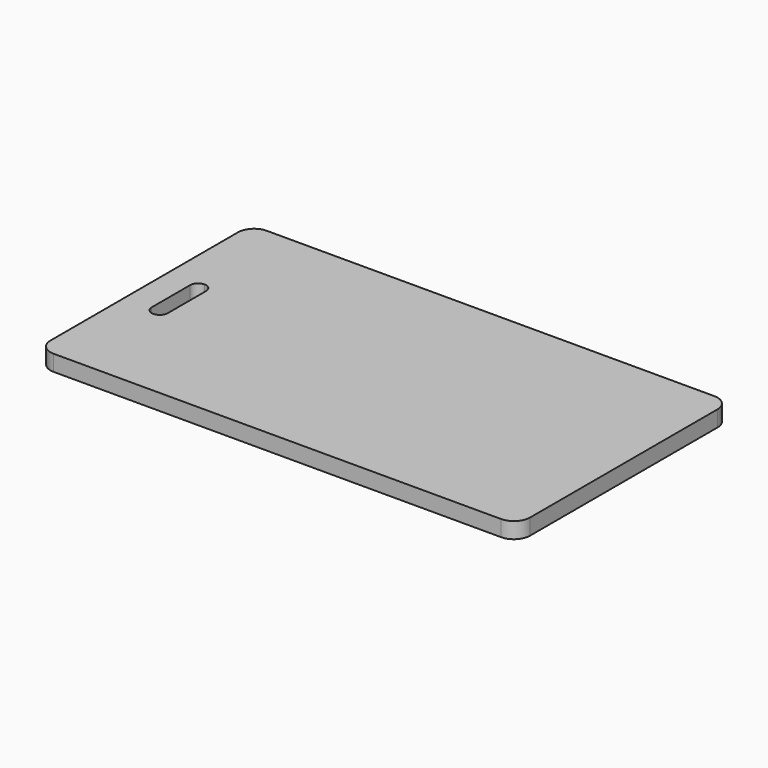
from build123d import *

# Parameters (mm, degrees)
F0_W     = 3
F0_H     = 12
F1_DEPTH = 3
F2_R     = 1.49999


# Not quite as in the source:
# - a fillet or chamfer is up to 0.001 mm smaller than in the source, because OpenCascade refuses the exact size
# - a feature of the source that left no trace in its solid (it failed there, or was rolled back) is left out


with BuildPart() as f1:
    # F0 (on Top) → F1 (new body)
    with BuildSketch(Plane.XY):
        with BuildLine():
            ThreePointArc((0, 3), (0.8786796564, 0.8786796564), (3, 0))
            Line((3, 0), (87, 0))
            ThreePointArc((87, 0), (89.1213203436, 0.8786796564), (90, 3))
            Line((90, 3), (90, 47))
            ThreePointArc((90, 47), (89.1213203436, 49.1213203436), (87, 50))
            Line((87, 50), (3, 50))
            ThreePointArc((3, 50), (0.8786796564, 49.1213203436), (0, 47))
            Line((0, 47), (0, 3))
        make_face()
        with Locations((6.5, 25)):
            Rectangle(F0_W, F0_H, mode=Mode.SUBTRACT)
    extrude(amount=F1_DEPTH)

    # F2 (radius 1.5 in the source; OpenCascade refuses exactly that, so slightly less here)
    f2_edges = [f1.edges().sort_by_distance(p)[0] for p in [
        (5, 31, 1.5),
        (8, 31, 1.5),
        (5, 19, 1.5),
        (8, 19, 1.5),
    ]]
    fillet(f2_edges, radius=F2_R)


solid = f1.part
